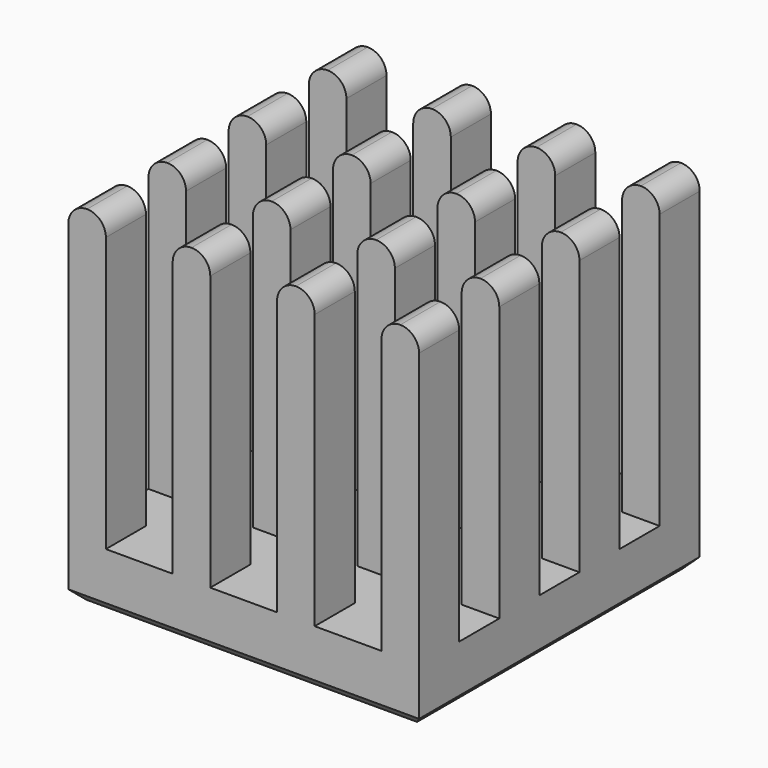
from build123d import *

# Parameters (mm, degrees)
F0_W     = 14
F0_H     = 14
F1_DEPTH = 2.3
F2_W     = 1.5
F2_H     = 2
F3_DEPTH = 11.7
F4_SIZE  = 0.4
F5_R     = 0.74999


# Not quite as in the source:
# - a fillet or chamfer is up to 0.001 mm smaller than in the source, because OpenCascade refuses the exact size


with BuildPart() as f1:
    # F0 (on Top) → F1 (new body)
    with BuildSketch(Plane.XY):
        with Locations((7, 7)):
            Rectangle(F0_W, F0_H)
    extrude(amount=F1_DEPTH)

    # F2 (on face) → F3 (join)
    with BuildSketch(Plane.XY.offset(2.3)):
        with Locations((0.75, 13)):
            Rectangle(F2_W, F2_H)
        with Locations((0.75, 1)):
            Rectangle(F2_W, F2_H)
        with Locations((13.25, 13)):
            Rectangle(F2_W, F2_H)
        with Locations((13.25, 1)):
            Rectangle(F2_W, F2_H)
        with Locations((0.75, 9)):
            Rectangle(F2_W, F2_H)
        with Locations((0.75, 5)):
            Rectangle(F2_W, F2_H)
        with Locations((13.25, 9)):
            Rectangle(F2_W, F2_H)
        with Locations((13.25, 5)):
            Rectangle(F2_W, F2_H)
        with Locations((4.9166666667, 9)):
            Rectangle(F2_W, F2_H)
        with Locations((9.0833333333, 9)):
            Rectangle(F2_W, F2_H)
        with Locations((4.9166666667, 13)):
            Rectangle(F2_W, F2_H)
        with Locations((9.0833333333, 13)):
            Rectangle(F2_W, F2_H)
        with Locations((4.9166666667, 5)):
            Rectangle(F2_W, F2_H)
        with Locations((9.0833333333, 5)):
            Rectangle(F2_W, F2_H)
        with Locations((4.9166666667, 1)):
            Rectangle(F2_W, F2_H)
        with Locations((9.0833333333, 1)):
            Rectangle(F2_W, F2_H)
    extrude(amount=F3_DEPTH)

    # F4
    f4_edges = [f1.edges().sort_by_distance(p)[0] for p in [
        (7, 0, 0),
        (0, 7, 0),
        (14, 7, 0),
        (7, 14, 0),
    ]]
    chamfer(f4_edges, length=F4_SIZE)

    # F5 (radius 0.75 in the source; OpenCascade refuses exactly that, so slightly less here)
    f5_edges = [f1.edges().sort_by_distance(p)[0] for p in [
        (14, 13, 14),
        (12.5, 13, 14),
        (9.833333, 13, 14),
        (8.333333, 13, 14),
        (5.666667, 13, 14),
        (4.166667, 13, 14),
        (1.5, 13, 14),
        (0, 13, 14),
        (0, 9, 14),
        (1.5, 9, 14),
        (4.166667, 9, 14),
        (5.666667, 9, 14),
        (8.333333, 9, 14),
        (9.833333, 9, 14),
        (12.5, 9, 14),
        (14, 9, 14),
        (14, 5, 14),
        (12.5, 5, 14),
        (9.833333, 5, 14),
        (8.333333, 5, 14),
        (5.666667, 5, 14),
        (4.166667, 5, 14),
        (1.5, 5, 14),
        (0, 5, 14),
        (0, 1, 14),
        (1.5, 1, 14),
        (4.166667, 1, 14),
        (5.666667, 1, 14),
        (8.333333, 1, 14),
        (9.833333, 1, 14),
        (12.5, 1, 14),
        (14, 1, 14),
    ]]
    fillet(f5_edges, radius=F5_R)


solid = f1.part
